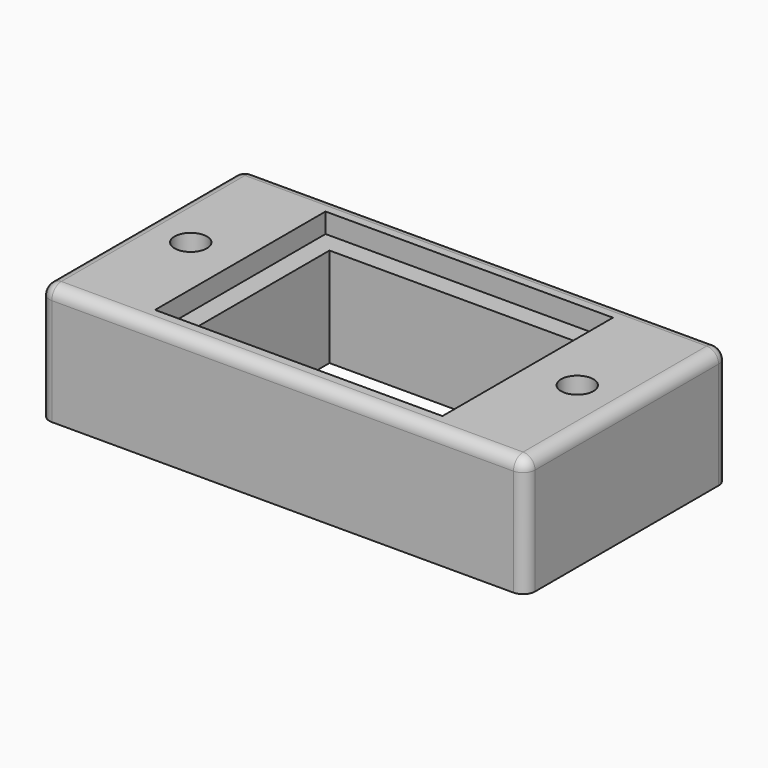
from build123d import *

# Parameters (mm, degrees)
F0_W     = 49
F0_H     = 25.5652221807
F1_DEPTH = 12
F2_W     = 29
F2_H     = 21.5
F3_DEPTH = 2
F4_W     = 25
F4_H     = 17.5
F5_DEPTH = 12
F7_D     = 3.2639
F8_R     = 1.207
F9_R     = 1.207
F10_R    = 1.207
F11_R    = 1.207


# Not quite as in the source:
# - a feature names something its author has since deleted; it is built from what else it names


with BuildPart() as f1:
    # F0 (on Top) → F1 (new body)
    with BuildSketch(Plane.XY):
        Rectangle(F0_W, F0_H)
    extrude(amount=-F1_DEPTH)

    # F2 (on face) → F3 (cut)
    with BuildSketch(Plane.XY):
        Rectangle(F2_W, F2_H)
    extrude(amount=-F3_DEPTH, mode=Mode.SUBTRACT)

    # F4 (on Top) → F5 (cut)
    with BuildSketch(Plane.XY):
        Rectangle(F4_W, F4_H)
    extrude(amount=-F5_DEPTH, mode=Mode.SUBTRACT)

    # F7 (through all)
    with Locations(Plane.XY):
        with Locations((-19.5, 0), (19.5, 0)):
            Hole(F7_D / 2)

    # F8
    f8_edges = [f1.edges().sort_by_distance(p)[0] for p in [
        (0, -12.782611, 0),
    ]]
    fillet(f8_edges, radius=F8_R)

    # F9
    f9_edges = [f1.edges().sort_by_distance(p)[0] for p in [
        (24.5, 0.6035, 0),
    ]]
    fillet(f9_edges, radius=F9_R)

    # F10
    f10_edges = [f1.edges().sort_by_distance(p)[0] for p in [
        (-24.5, 0.6035, 0),
    ]]
    fillet(f10_edges, radius=F10_R)

    # F11
    f11_edges = [f1.edges().sort_by_distance(p)[0] for p in [
        (0, 12.782611, 0),
    ]]
    fillet(f11_edges, radius=F11_R)


solid = f1.part
